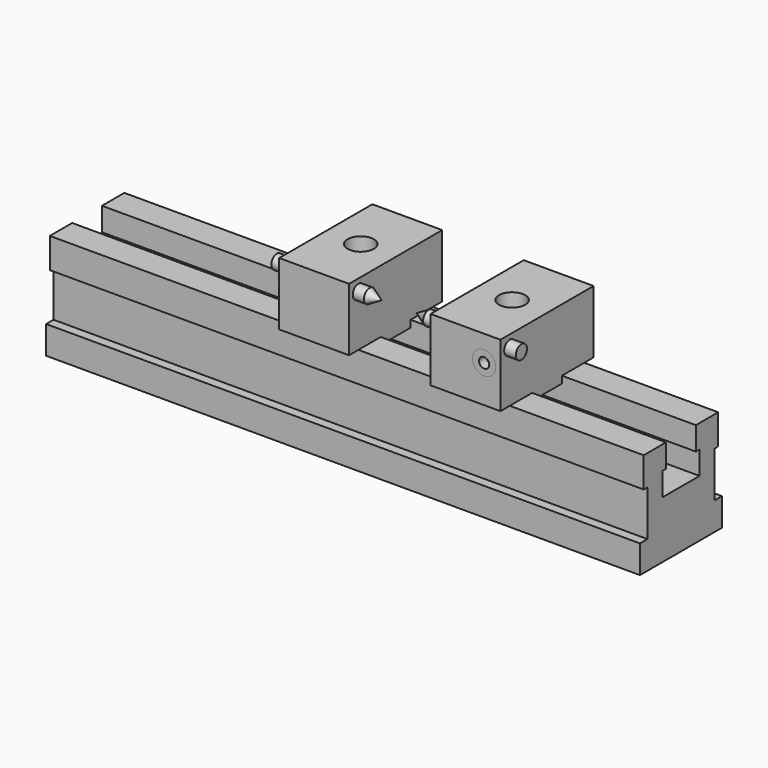
from build123d import *

# Parameters (mm, degrees)
F1_DEPTH        = 127.5
F5_DEPTH        = 30
F7_DEPTH        = 30
F8_R            = 3
F9_DEPTH        = 197.501
F10_R           = 3
F11_DEPTH       = 132.501
F14_D           = 6.6
F14_CBORE_D     = 11.25
F14_CBORE_DEPTH = 6
F15_D           = 6.6
F15_CBORE_D     = 11.25
F15_CBORE_DEPTH = 6
F20_R           = 5
F20_R_2         = 2
F21_DEPTH       = 20
F22_DEPTH       = 15
F23_D           = 4.4
F24_DEPTH       = 202.501
F25_W           = 10
F25_H           = 2
F26_DEPTH       = 66.501


with BuildPart() as f1:
    # F0 (on Right) → F1 (new body, symmetric)
    with BuildSketch(Plane.YZ):
        Polygon((-22, 0), (0, 0), (0, 24.5), (-10, 24.5), (-10, 34.5), (-8, 34.5), (-8, 41.5), (-8, 44.5), (-20, 44.5), (-20, 31.5588298937), (-18, 31.5588298937), (-18, 12), (-22, 12), align=None)
        Polygon((0, 24.5), (0, 0), (22, 0), (22, 12), (18, 12), (18, 31.5588298937), (20, 31.5588298937), (20, 44.5), (8, 44.5), (8, 41.5), (8, 34.5), (10, 34.5), (10, 24.5), align=None)
    extrude(amount=F1_DEPTH, both=True)

    # F10 (on face) → F11 (cut, through all)
    with BuildSketch(Plane.YZ.offset(5)):
        with Locations((-20, 66.5)):
            Circle(F10_R)
    extrude(amount=-F11_DEPTH, mode=Mode.SUBTRACT)


with BuildPart() as f5:
    # F4 (on offset) → F5 (new body)
    with BuildSketch(Plane.YZ.offset(40)):
        Polygon((-25, 71.5), (-25, 44.5), (-8, 44.5), (-8, 41.5), (8, 41.5), (8, 44.5), (25, 44.5), (25, 71.5), align=None)
    extrude(amount=F5_DEPTH)


with BuildPart() as f7:
    # F6 (on offset) → F7 (new body)
    with BuildSketch(Plane.YZ.offset(-25)):
        Polygon((-8, 41.5), (8, 41.5), (8, 44.5), (20, 44.5), (25, 44.5), (25, 71.5), (-25, 71.5), (-25, 44.5), (-20, 44.5), (-8, 44.5), align=None)
    extrude(amount=F7_DEPTH)


with BuildPart() as f9_tool:
    # F8 (on face) → F9 (new body, through all)
    with BuildSketch(Plane.YZ.offset(70)):
        with Locations((-20, 66.5)):
            Circle(F8_R)
    extrude(amount=-F9_DEPTH)


with BuildPart() as f5_1:
    add(f5.part)

    # F9: cut by f9_tool
    add(f9_tool.part, mode=Mode.SUBTRACT)

    # F15 (through all)
    with Locations(Plane.XY.offset(71.5)):
        with Locations((55, 0)):
            CounterBoreHole(F15_D / 2, F15_CBORE_D / 2, F15_CBORE_DEPTH)

    # F20 (on face) → F21 (cut)
    with BuildSketch(Plane.XZ.offset(25)):
        with Locations((63, 60.5)):
            Circle(F20_R)
        with Locations((63, 60.5)):
            Circle(F20_R_2, mode=Mode.SUBTRACT)
        with Locations((63, 60.5)):
            Circle(F20_R_2)
    extrude(amount=-F21_DEPTH, mode=Mode.SUBTRACT)


with BuildPart() as f7_1:
    add(f7.part)

    # F9: cut by f9_tool
    add(f9_tool.part, mode=Mode.SUBTRACT)

    # F14 (through all)
    with Locations(Plane.XY.offset(71.5)):
        with Locations((-10, 0)):
            CounterBoreHole(F14_D / 2, F14_CBORE_D / 2, F14_CBORE_DEPTH)


with BuildPart() as f18:
    # F17 (on offset) → F18 (revolve)
    with BuildSketch(Plane.XY.offset(66.5)):
        Polygon((75, -20), (30, -20), (35.1961524227, -23), (75, -23), align=None)
    revolve(axis=Axis((28.5532526373, -20, 66.5), (1, 0, 0)))


with BuildPart() as f19:
    # F17 (on offset) → F19 (revolve)
    with BuildSketch(Plane.XY.offset(66.5)):
        Polygon((15, -20), (-30, -20), (-30, -23), (9.8038475773, -23), align=None)
    revolve(axis=Axis((-7.5, -20, 66.5), (1, 0, 0)))


with BuildPart() as f22:
    # F20 (on face) → F22 (new body)
    with BuildSketch(Plane.XZ.offset(25)):
        with Locations((63, 60.5)):
            Circle(F20_R)
        with Locations((63, 60.5)):
            Circle(F20_R_2, mode=Mode.SUBTRACT)
        with Locations((63, 60.5)):
            Circle(F20_R_2)
    extrude(amount=-F22_DEPTH)

    # F23 (through all)
    with Locations(Plane.XZ.offset(25)):
        with Locations((63, 60.5)):
            Hole(F23_D / 2)

    # F24 (cut, through all): a face of the model
    f24_faces = [f18.part.faces().sort_by_distance(p)[0] for p in [
        (75, -20, 66.5),
    ]]
    extrude(f24_faces, amount=-F24_DEPTH, mode=Mode.SUBTRACT)

    # F25 (on offset) → F26 (cut, through all)
    with BuildSketch(Plane.XY.offset(66.5)):
        with Locations((63, -20)):
            Rectangle(F25_W, F25_H)
    extrude(amount=-F26_DEPTH, mode=Mode.SUBTRACT)


solid = Compound([f1.part, f5_1.part, f7_1.part, f18.part, f19.part, f22.part])
